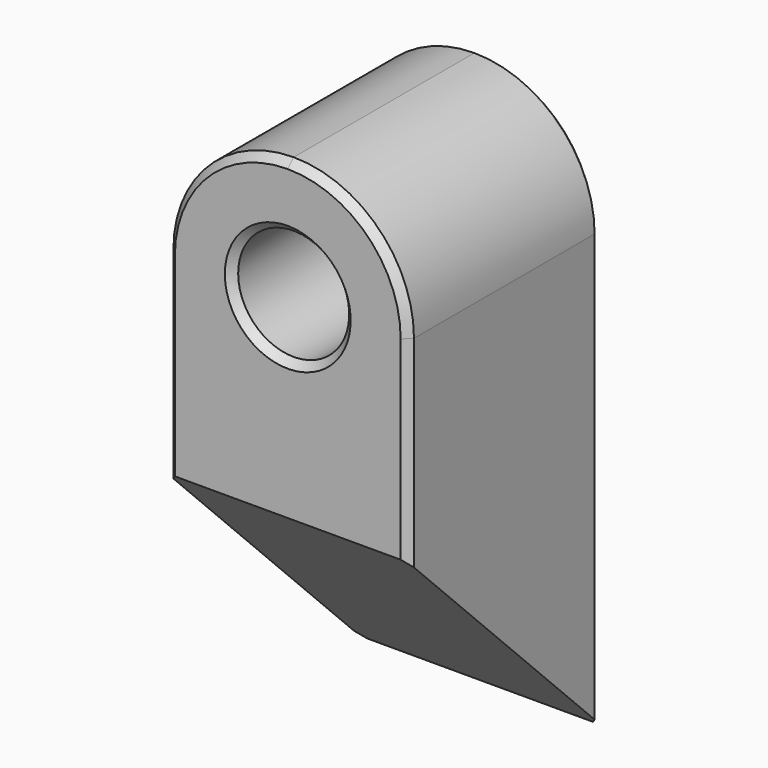
from build123d import *

# Parameters (mm, degrees)
F0_W     = 13
F0_H     = 13
F1_DEPTH = 30
F2_SIZE  = 12.99999
F3_R     = 6.49999
F4_R     = 3
F5_DEPTH = 25
F6_SIZE  = 0.4


# Not quite as in the source:
# - a fillet or chamfer is up to 0.001 mm smaller than in the source, because OpenCascade refuses the exact size


with BuildPart() as f1:
    # F0 (on Top) → F1 (new body)
    with BuildSketch(Plane.XY):
        Rectangle(F0_W, F0_H)
    extrude(amount=F1_DEPTH)

    # F2 (size 13 in the source; OpenCascade refuses exactly that, so slightly less here)
    f2_edges = [f1.edges().sort_by_distance(p)[0] for p in [
        (0, -6.5, 0),
    ]]
    chamfer(f2_edges, length=F2_SIZE)

    # F3 (radius 6.5 in the source; OpenCascade refuses exactly that, so slightly less here)
    f3_edges = [f1.edges().sort_by_distance(p)[0] for p in [
        (6.5, 0, 30),
        (-6.5, 0, 30),
    ]]
    fillet(f3_edges, radius=F3_R)

    # F4 (on face) → F5 (cut)
    with BuildSketch(Plane(origin=(0, 6.5, 0), x_dir=(-1, 0, 0), z_dir=(0, 1, 0))):
        with Locations((0, 23.5)):
            Circle(F4_R)
    extrude(amount=-F5_DEPTH, mode=Mode.SUBTRACT)

    # F6
    f6_edges = [f1.edges().sort_by_distance(p)[0] for p in [
        (4.596197, 6.5, 28.096197),
        (4.596197, -6.5, 28.096197),
        (3, 6.5, 23.5),
        (3, -6.5, 23.5),
    ]]
    chamfer(f6_edges, length=F6_SIZE)


solid = f1.part
